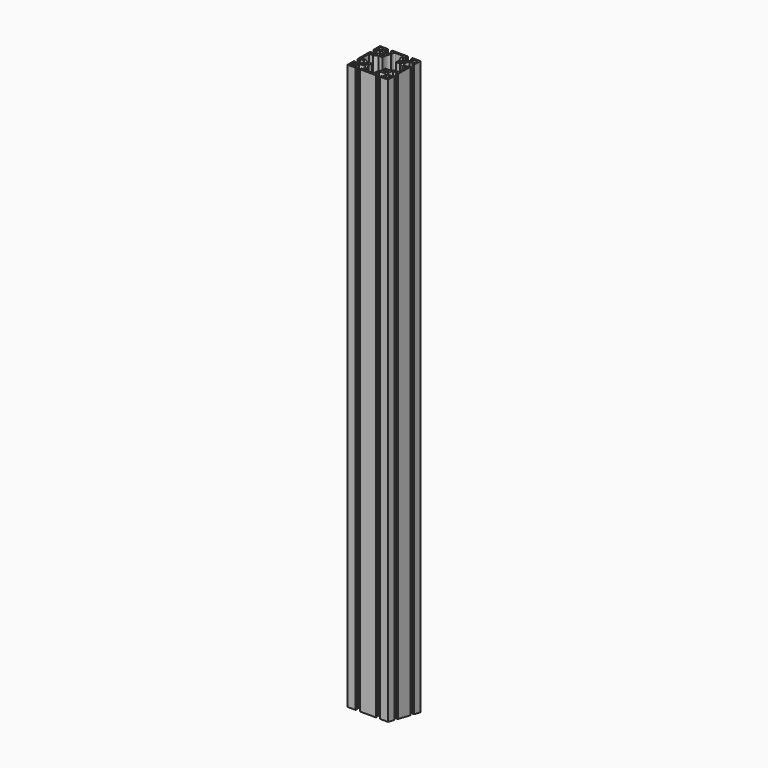
from build123d import *

# Parameters (mm, degrees)
F0_R          = 3
F0_R_2        = 2.5
F1_DEPTH      = 850
F2_R          = 2
F3_R          = 7
F5_DEPTH      = 30
F5_DEPTH_BACK = 30


# Not quite as in the source:
# - a feature names something its author has since deleted; it is built from what else it names


with BuildPart() as f1:
    # F0 (on Top) → F1 (new body)
    with BuildSketch(Plane.XY):
        with BuildLine():
            Line((18.15, -30), (30, -30))
            Line((30, -30), (30, -18.15))
            Line((30, -18.15), (27.5, -18.15))
            Line((27.5, -18.15), (27.5, -20.15))
            Line((27.5, -20.15), (21.5477069044, -20.15))
            ThreePointArc((21.5477069044, -20.15), (19.5, -15), (21.5477069044, -9.85))
            Line((21.5477069044, -9.85), (27.5, -9.85))
            Line((27.5, -9.85), (27.5, -11.85))
            Line((27.5, -11.85), (30, -11.85))
            Line((30, -11.85), (30, 11.85))
            Line((30, 11.85), (27.5, 11.85))
            Line((27.5, 11.85), (27.5, 9.85))
            Line((27.5, 9.85), (21.5477069044, 9.85))
            ThreePointArc((21.5477069044, 9.85), (19.5, 15), (21.5477069044, 20.15))
            Line((21.5477069044, 20.15), (27.5, 20.15))
            Line((27.5, 20.15), (27.5, 18.15))
            Line((27.5, 18.15), (30, 18.15))
            Line((30, 18.15), (30, 30))
            Line((30, 30), (18.15, 30))
            Line((18.15, 30), (18.15, 27.5))
            Line((18.15, 27.5), (20.15, 27.5))
            Line((20.15, 27.5), (20.15, 21.5477069044))
            ThreePointArc((20.15, 21.5477069044), (15, 19.5), (9.85, 21.5477069044))
            Line((9.85, 21.5477069044), (9.85, 27.5))
            Line((9.85, 27.5), (11.85, 27.5))
            Line((11.85, 27.5), (11.85, 30))
            Line((11.85, 30), (-11.85, 30))
            Line((-11.85, 30), (-11.85, 27.5))
            Line((-11.85, 27.5), (-9.85, 27.5))
            Line((-9.85, 27.5), (-9.85, 21.5477069044))
            ThreePointArc((-9.85, 21.5477069044), (-15, 19.5), (-20.15, 21.5477069044))
            Line((-20.15, 21.5477069044), (-20.15, 27.5))
            Line((-20.15, 27.5), (-18.15, 27.5))
            Line((-18.15, 27.5), (-18.15, 30))
            Line((-18.15, 30), (-30, 30))
            Line((-30, 30), (-30, 18.15))
            Line((-30, 18.15), (-27.5, 18.15))
            Line((-27.5, 18.15), (-27.5, 20.15))
            Line((-27.5, 20.15), (-21.5477069044, 20.15))
            ThreePointArc((-21.5477069044, 20.15), (-19.5, 15), (-21.5477069044, 9.85))
            Line((-21.5477069044, 9.85), (-27.5, 9.85))
            Line((-27.5, 9.85), (-27.5, 11.85))
            Line((-27.5, 11.85), (-30, 11.85))
            Line((-30, 11.85), (-30, -11.85))
            Line((-30, -11.85), (-27.5, -11.85))
            Line((-27.5, -11.85), (-27.5, -9.85))
            Line((-27.5, -9.85), (-21.5477069044, -9.85))
            ThreePointArc((-21.5477069044, -9.85), (-19.5, -15), (-21.5477069044, -20.15))
            Line((-21.5477069044, -20.15), (-27.5, -20.15))
            Line((-27.5, -20.15), (-27.5, -18.15))
            Line((-27.5, -18.15), (-30, -18.15))
            Line((-30, -18.15), (-30, -30))
            Line((-30, -30), (-18.15, -30))
            Line((-18.15, -30), (-18.15, -27.5))
            Line((-18.15, -27.5), (-20.15, -27.5))
            Line((-20.15, -27.5), (-20.15, -21.5477069044))
            ThreePointArc((-20.15, -21.5477069044), (-15, -19.5), (-9.85, -21.5477069044))
            Line((-9.85, -21.5477069044), (-9.85, -27.5))
            Line((-9.85, -27.5), (-11.85, -27.5))
            Line((-11.85, -27.5), (-11.85, -30))
            Line((-11.85, -30), (11.85, -30))
            Line((11.85, -30), (11.85, -27.5))
            Line((11.85, -27.5), (9.85, -27.5))
            Line((9.85, -27.5), (9.85, -21.5477069044))
            ThreePointArc((9.85, -21.5477069044), (15, -19.5), (20.15, -21.5477069044))
            Line((20.15, -21.5477069044), (20.15, -27.5))
            Line((20.15, -27.5), (18.15, -27.5))
            Line((18.15, -27.5), (18.15, -30))
        make_face()
        with Locations((-25, -25)):
            Circle(F0_R, mode=Mode.SUBTRACT)
        with Locations((-15, -15)):
            Circle(F0_R_2, mode=Mode.SUBTRACT)
        with Locations((25, -25)):
            Circle(F0_R, mode=Mode.SUBTRACT)
        with Locations((15, -15)):
            Circle(F0_R_2, mode=Mode.SUBTRACT)
        with Locations((-25, 25)):
            Circle(F0_R, mode=Mode.SUBTRACT)
        with Locations((-15, 15)):
            Circle(F0_R_2, mode=Mode.SUBTRACT)
        Polygon((-7, 22), (-7, 27.5), (0, 27.5), (7, 27.5), (7, 22), (10, 16), (10, 10), (16, 10), (22, 7), (27.5, 7), (27.5, 0), (27.5, -7), (22, -7), (16, -10), (10, -10), (10, -16), (7, -22), (7, -27.5), (0, -27.5), (-7, -27.5), (-7, -22), (-10, -16), (-10, -10), (-16, -10), (-22, -7), (-27.5, -7), (-27.5, 0), (-27.5, 7), (-22, 7), (-16, 10), (-10, 10), (-10, 16), align=None, mode=Mode.SUBTRACT)
        with Locations((15, 15)):
            Circle(F0_R_2, mode=Mode.SUBTRACT)
        with Locations((25, 25)):
            Circle(F0_R, mode=Mode.SUBTRACT)
    extrude(amount=F1_DEPTH)

    # F2
    f2_edges = [f1.edges().sort_by_distance(p)[0] for p in [
        (-7, 27.5, 425),
        (7, 27.5, 425),
    ]]
    fillet(f2_edges, radius=F2_R)

    # F3
    f3_edges = [f1.edges().sort_by_distance(p)[0] for p in [
        (-10, 16, 425),
        (10, 16, 425),
    ]]
    fillet(f3_edges, radius=F3_R)

    # F4 (on Right) → F5 (cut, two sides)
    with BuildSketch(Plane.YZ) as f5_sk:
        Polygon((-164.2855995683, 38.6458085579), (-188.5911429791, -83.5464097089), (5.6944565892, -122.1922182668), (30, 0), align=None)
    extrude(amount=F5_DEPTH, mode=Mode.SUBTRACT)
    extrude(f5_sk.sketch, amount=-F5_DEPTH_BACK, mode=Mode.SUBTRACT)


solid = f1.part
